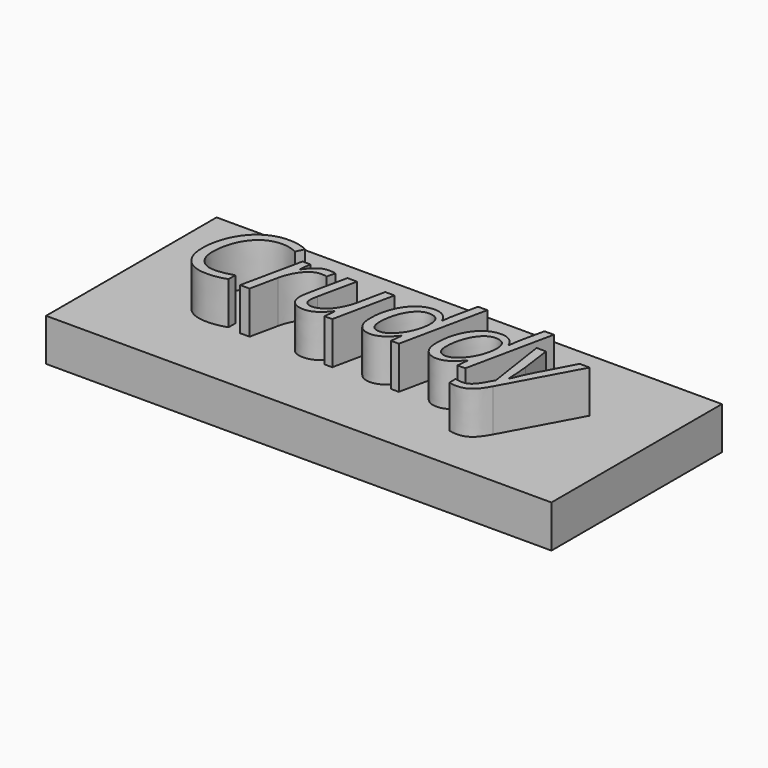
from build123d import *

# Parameters (mm, degrees)
F0_W         = 75.7083892822
F0_H         = 31.9275297225
F1_DEPTH     = 6.35
F2_TEXT_SIZE = 17.2512502306
F3_DEPTH     = 12.7


# Not quite as in the source:
# - Text() gives the source's letters only with a copy of the font that has no kerning and outlines rounded to 1/6400 em; it was checked with that copy


with BuildPart() as f1:
    # F0 (on Top) → F1 (new body)
    with BuildSketch(Plane.XY):
        Rectangle(F0_W, F0_H)
    extrude(amount=F1_DEPTH)

    # F2 (on Top) → F3 (join)
    with BuildSketch(Plane.XY):
        with Locations((-27.9605481774, -5.231582094)):
            Text('Cruddy', F2_TEXT_SIZE, font='Open Sans', font_style=FontStyle.ITALIC, text_align=(TextAlign.LEFT, TextAlign.BOTTOM))
    extrude(amount=F3_DEPTH)


solid = f1.part
